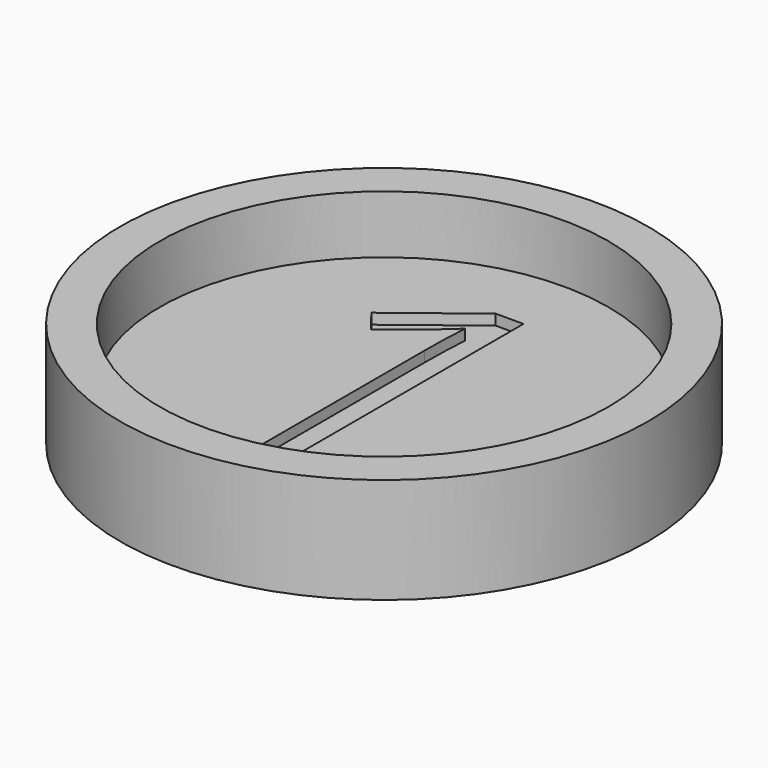
from build123d import *

# Parameters (mm, degrees)
F0_R         = 25
F1_DEPTH     = 10
F2_R         = 21.25
F3_DEPTH     = 5.5
F4_TEXT_SIZE = 38.4976143121
F5_DEPTH     = 1


# Not quite as in the source:
# - Text() gives the source's letters only with a copy of the font that has no kerning and outlines rounded to 1/6400 em; it was checked with that copy


with BuildPart() as f1:
    # F0 (on Top) → F1 (new body)
    with BuildSketch(Plane.XY):
        Circle(F0_R)
    extrude(amount=F1_DEPTH)

    # F2 (on face) → F3 (cut)
    with BuildSketch(Plane.XY.offset(10)):
        Circle(F2_R)
    extrude(amount=-F3_DEPTH, mode=Mode.SUBTRACT)

    # F4 (on face) → F5 (cut)
    with BuildSketch(Plane.XY.offset(4.5)):
        with Locations((-11.9987494515, -12.784788385)):
            Text('1', F4_TEXT_SIZE, font='Open Sans', text_align=(TextAlign.LEFT, TextAlign.BOTTOM))
    extrude(amount=-F5_DEPTH, mode=Mode.SUBTRACT)


solid = f1.part
